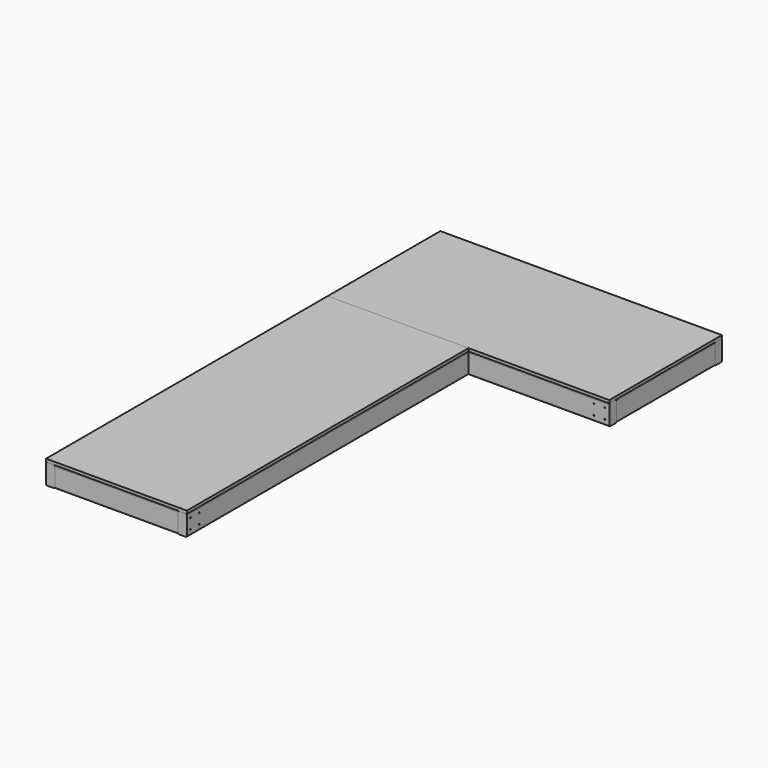
from build123d import *

# Parameters (mm, degrees)
F1_DEPTH  = 12.7
F2_W      = 609.6
F2_H      = 1524
F3_DEPTH  = 12.7
F5_DEPTH  = 88.9
F4_W      = 533.4
F4_H      = 38.1
F6_DEPTH  = 88.9
F7_DEPTH  = 88.9
F8_DEPTH  = 88.9
F9_DEPTH  = 88.9
F10_DEPTH = 88.9
F4_W_2    = 38.1
F4_H_2    = 533.4
F11_DEPTH = 88.9
F12_DEPTH = 88.9
F13_DEPTH = 88.9
F14_DEPTH = 88.9
F15_DEPTH = 88.9
F16_R     = 5.08
F16_2_R   = 5.08
F16_3_R   = 5.08
F16_4_R   = 5.08
F16_5_R   = 5.08
F16_6_R   = 5.08
F16_7_R   = 5.08
F16_8_R   = 5.08
F16_9_R   = 5.08
F16_10_R  = 5.08
F16_11_R  = 5.08
F17_R     = 2.38125
F19_DEPTH = 38.1
F18_R     = 2.38125
F20_DEPTH = 38.1
F21_R     = 2.38125
F22_DEPTH = 38.1
F23_R     = 2.38125
F24_DEPTH = 38.1


with BuildPart() as f1:
    # F0 (on Top) → F1 (new body)
    with BuildSketch(Plane.XY):
        Polygon((0, 609.6), (0, 0), (609.6, 0), (1219.2, 0), (1219.2, 609.6), align=None)
    extrude(amount=F1_DEPTH)


with BuildPart() as f3:
    # F2 (on Top) → F3 (new body)
    with BuildSketch(Plane.XY):
        with Locations((304.8, -762)):
            Rectangle(F2_W, F2_H)
    extrude(amount=F3_DEPTH)


with BuildPart() as f5:
    # F4 (on Top) → F5 (new body)
    with BuildSketch(Plane.XY):
        Polygon((38.1, 571.5), (38.1, 609.6), (0, 609.6), (0, -1524), (38.1, -1524), (38.1, -1485.9), (38.1, -1476.375), (38.1, -1438.275), (38.1, 254), (38.1, 292.1), (38.1, 301.625), (38.1, 339.725), (38.1, 523.875), (38.1, 561.975), align=None)
    extrude(amount=-F5_DEPTH)

    # F16
    f16_edges = [f5.edges().sort_by_distance(p)[0] for p in [
        (0, -457.2, -88.9),
        (38.1, -457.2, -88.9),
        (38.1, -457.2, 0),
        (0, -457.2, 0),
    ]]
    fillet(f16_edges, radius=F16_R)

    # F17 (on face) → F19 (cut)
    with BuildSketch(Plane(origin=(0, 0, 0), x_dir=(0, -1, 0), z_dir=(-1, 0, 0))):
        with Locations((-590.55, -22.225)):
            Circle(F17_R)
        with Locations((-590.55, -66.5618479609)):
            Circle(F17_R)
        with Locations((-542.925, -66.6410699844)):
            Circle(F17_R)
        with Locations((-542.925, -22.225)):
            Circle(F17_R)
        with Locations((-320.675, -22.225)):
            Circle(F17_R)
        with Locations((-320.675, -66.675)):
            Circle(F17_R)
        with Locations((-273.05, -22.225)):
            Circle(F17_R)
        with Locations((-273.05, -66.675)):
            Circle(F17_R)
        with Locations((1457.325, -66.675)):
            Circle(F17_R)
        with Locations((1457.325, -22.225)):
            Circle(F17_R)
        with Locations((1504.95, -22.225)):
            Circle(F17_R)
        with Locations((1504.95, -66.675)):
            Circle(F17_R)
    extrude(amount=-F19_DEPTH, mode=Mode.SUBTRACT)


with BuildPart() as f6:
    # F4 (on Top) → F6 (new body)
    with BuildSketch(Plane.XY):
        with Locations((304.8, -1504.95)):
            Rectangle(F4_W, F4_H)
    extrude(amount=-F6_DEPTH)

    # F16#3
    f16_3_edges = [f6.edges().sort_by_distance(p)[0] for p in [
        (304.8, -1485.9, 0),
        (304.8, -1524, 0),
        (304.8, -1485.9, -88.9),
        (304.8, -1524, -88.9),
    ]]
    fillet(f16_3_edges, radius=F16_3_R)


with BuildPart() as f7:
    # F4 (on Top) → F7 (new body)
    with BuildSketch(Plane.XY):
        Polygon((609.6, 571.5), (571.5, 571.5), (571.5, 561.975), (571.5, 523.875), (571.5, 339.725), (571.5, 301.625), (571.5, 292.1), (571.5, 254), (571.5, -1438.275), (571.5, -1476.375), (571.5, -1485.9), (571.5, -1524), (609.6, -1524), (609.6, 0), (609.6, 38.1), align=None)
    extrude(amount=-F7_DEPTH)

    # F16#2
    f16_2_edges = [f7.edges().sort_by_distance(p)[0] for p in [
        (571.5, -476.25, -88.9),
        (609.6, -476.25, -88.9),
        (571.5, -476.25, 0),
        (609.6, -476.25, 0),
    ]]
    fillet(f16_2_edges, radius=F16_2_R)

    # F18 (on face) → F20 (cut)
    with BuildSketch(Plane.YZ.offset(609.6)):
        with Locations((-1457.325, -22.225)):
            Circle(F18_R)
        with Locations((-1504.95, -22.225)):
            Circle(F18_R)
        with Locations((-1504.95, -66.675)):
            Circle(F18_R)
        with Locations((-1457.325, -66.675)):
            Circle(F18_R)
        with Locations((273.05, -22.225)):
            Circle(F18_R)
        with Locations((273.05, -66.675)):
            Circle(F18_R)
        with Locations((320.675, -22.225)):
            Circle(F18_R)
        with Locations((320.675, -66.675)):
            Circle(F18_R)
        with Locations((542.925, -22.225)):
            Circle(F18_R)
        with Locations((542.925, -66.675)):
            Circle(F18_R)
        with Locations((19.05, -22.225)):
            Circle(F18_R)
        with Locations((19.05, -66.675)):
            Circle(F18_R)
    extrude(amount=-F20_DEPTH, mode=Mode.SUBTRACT)


with BuildPart() as f8:
    # F4 (on Top) → F8 (new body)
    with BuildSketch(Plane.XY):
        Polygon((1219.2, 0), (1219.2, 38.1), (1181.1, 38.1), (1171.575, 38.1), (1133.475, 38.1), (609.6, 38.1), (609.6, 0), align=None)
    extrude(amount=-F8_DEPTH)

    # F16#5
    f16_5_edges = [f8.edges().sort_by_distance(p)[0] for p in [
        (914.4, 38.1, -88.9),
        (914.4, 0, -88.9),
        (914.4, 38.1, 0),
        (914.4, 0, 0),
    ]]
    fillet(f16_5_edges, radius=F16_5_R)

    # F21 (on face) → F22 (cut)
    with BuildSketch(Plane.XZ):
        with Locations((1200.15, -66.675)):
            Circle(F21_R)
        with Locations((1200.15, -22.225)):
            Circle(F21_R)
        with Locations((1152.525, -22.225)):
            Circle(F21_R)
        with Locations((1152.525, -66.675)):
            Circle(F21_R)
    extrude(amount=-F22_DEPTH, mode=Mode.SUBTRACT)


with BuildPart() as f9:
    # F4 (on Top) → F9 (new body)
    with BuildSketch(Plane.XY):
        with Locations((304.8, 273.05)):
            Rectangle(F4_W, F4_H)
    extrude(amount=-F9_DEPTH)

    # F16#4
    f16_4_edges = [f9.edges().sort_by_distance(p)[0] for p in [
        (304.8, 254, -88.9),
        (304.8, 292.1, 0),
        (304.8, 292.1, -88.9),
        (304.8, 254, 0),
    ]]
    fillet(f16_4_edges, radius=F16_4_R)


with BuildPart() as f10:
    # F4 (on Top) → F10 (new body)
    with BuildSketch(Plane.XY):
        Polygon((1219.2, 609.6), (38.1, 609.6), (38.1, 571.5), (571.5, 571.5), (609.6, 571.5), (1133.475, 571.5), (1171.575, 571.5), (1181.1, 571.5), (1219.2, 571.5), align=None)
    extrude(amount=-F10_DEPTH)

    # F16#7
    f16_7_edges = [f10.edges().sort_by_distance(p)[0] for p in [
        (628.65, 571.5, -88.9),
        (628.65, 609.6, -88.9),
        (628.65, 609.6, 0),
        (628.65, 571.5, 0),
    ]]
    fillet(f16_7_edges, radius=F16_7_R)

    # F23 (on face) → F24 (cut)
    with BuildSketch(Plane(origin=(0, 609.6, 0), x_dir=(-1, 0, 0), z_dir=(0, 1, 0))):
        with Locations((-1200.15, -22.225)):
            Circle(F23_R)
        with Locations((-1200.15, -66.675)):
            Circle(F23_R)
        with Locations((-1152.525, -22.225)):
            Circle(F23_R)
        with Locations((-1152.525, -66.675)):
            Circle(F23_R)
    extrude(amount=-F24_DEPTH, mode=Mode.SUBTRACT)


with BuildPart() as f11:
    # F4 (on Top) → F11 (new body)
    with BuildSketch(Plane.XY):
        with Locations((1200.15, 304.8)):
            Rectangle(F4_W_2, F4_H_2)
    extrude(amount=-F11_DEPTH)

    # F16#6
    f16_6_edges = [f11.edges().sort_by_distance(p)[0] for p in [
        (1219.2, 304.8, -88.9),
        (1181.1, 304.8, -88.9),
        (1181.1, 304.8, 0),
        (1219.2, 304.8, 0),
    ]]
    fillet(f16_6_edges, radius=F16_6_R)


with BuildPart() as f12:
    # F4 (on Top) → F12 (new body)
    with BuildSketch(Plane.XY):
        with Locations((304.8, 320.675)):
            Rectangle(F4_W, F4_H)
    extrude(amount=-F12_DEPTH)

    # F16#8
    f16_8_edges = [f12.edges().sort_by_distance(p)[0] for p in [
        (304.8, 339.725, -88.9),
        (304.8, 301.625, -88.9),
        (304.8, 339.725, 0),
        (304.8, 301.625, 0),
    ]]
    fillet(f16_8_edges, radius=F16_8_R)


with BuildPart() as f13:
    # F4 (on Top) → F13 (new body)
    with BuildSketch(Plane.XY):
        with Locations((304.8, -1457.325)):
            Rectangle(F4_W, F4_H)
    extrude(amount=-F13_DEPTH)

    # F16#10
    f16_10_edges = [f13.edges().sort_by_distance(p)[0] for p in [
        (304.8, -1438.275, -88.9),
        (304.8, -1476.375, -88.9),
        (304.8, -1476.375, 0),
        (304.8, -1438.275, 0),
    ]]
    fillet(f16_10_edges, radius=F16_10_R)


with BuildPart() as f14:
    # F4 (on Top) → F14 (new body)
    with BuildSketch(Plane.XY):
        with Locations((304.8, 542.925)):
            Rectangle(F4_W, F4_H)
    extrude(amount=-F14_DEPTH)

    # F16#9
    f16_9_edges = [f14.edges().sort_by_distance(p)[0] for p in [
        (304.8, 523.875, -88.9),
        (304.8, 561.975, -88.9),
        (304.8, 523.875, 0),
        (304.8, 561.975, 0),
    ]]
    fillet(f16_9_edges, radius=F16_9_R)


with BuildPart() as f15:
    # F4 (on Top) → F15 (new body)
    with BuildSketch(Plane.XY):
        with Locations((1152.525, 304.8)):
            Rectangle(F4_W_2, F4_H_2)
    extrude(amount=-F15_DEPTH)

    # F16#11
    f16_11_edges = [f15.edges().sort_by_distance(p)[0] for p in [
        (1133.475, 304.8, -88.9),
        (1171.575, 304.8, -88.9),
        (1171.575, 304.8, 0),
        (1133.475, 304.8, 0),
    ]]
    fillet(f16_11_edges, radius=F16_11_R)


solid = Compound([f1.part, f3.part, f5.part, f6.part, f7.part, f8.part, f9.part, f10.part, f11.part, f12.part, f13.part, f14.part, f15.part])
